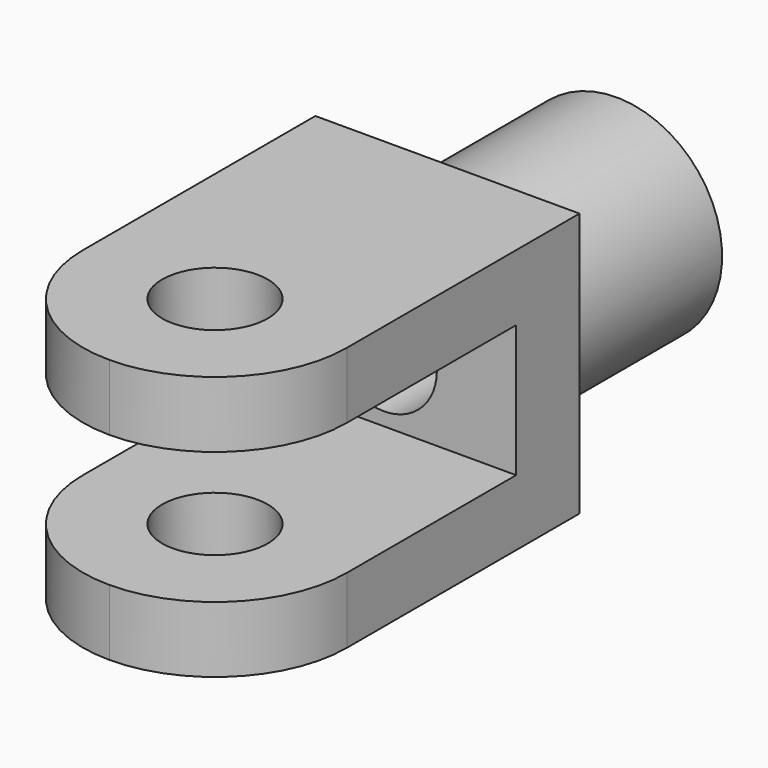
from build123d import *

# Parameters (mm, degrees)
F0_W     = 50
F0_H     = 50
F1_DEPTH = 7.5
F2_W     = 50
F2_H     = 12.5
F3_DEPTH = 65
F5_D     = 20
F6_R     = 25
F7_R     = 24.99999
F8_R     = 20
F9_DEPTH = 40
F11_D    = 20


# Not quite as in the source:
# - a fillet or chamfer is up to 0.001 mm smaller than in the source, because OpenCascade refuses the exact size


with BuildPart() as f1:
    # F0 (on Front) → F1 (new body, symmetric)
    with BuildSketch(Plane.XZ):
        Rectangle(F0_W, F0_H)
    extrude(amount=F1_DEPTH, both=True)

    # F2 (on face) → F3 (join)
    with BuildSketch(Plane.XZ.offset(7.5)):
        with Locations((0, -18.75)):
            Rectangle(F2_W, F2_H)
        with Locations((0, 18.75)):
            Rectangle(F2_W, F2_H)
    extrude(amount=F3_DEPTH)

    # F5 (through all)
    with Locations(Plane.XY.offset(25)):
        with Locations((0, -47.5)):
            Hole(F5_D / 2)

    # F6
    f6_edges = [f1.edges().sort_by_distance(p)[0] for p in [
        (-25, -72.5, -18.75),
    ]]
    fillet(f6_edges, radius=F6_R)

    # F7 (radius 25 in the source; OpenCascade refuses exactly that, so slightly less here)
    f7_edges = [f1.edges().sort_by_distance(p)[0] for p in [
        (25, -72.5, 18.75),
        (25, -72.5, -18.75),
        (-25, -72.5, 18.75),
    ]]
    fillet(f7_edges, radius=F7_R)

    # F8 (on face) → F9 (join)
    with BuildSketch(Plane(origin=(0, 7.5, 0), x_dir=(-1, 0, 0), z_dir=(0, 1, 0))):
        Circle(F8_R)
    extrude(amount=F9_DEPTH)

    # F11 (through all)
    with Locations(Plane(origin=(0, 47.5, 0), x_dir=(-1, 0, 0), z_dir=(0, 1, 0))):
        with Locations((0, 0)):
            Hole(F11_D / 2)


solid = f1.part
